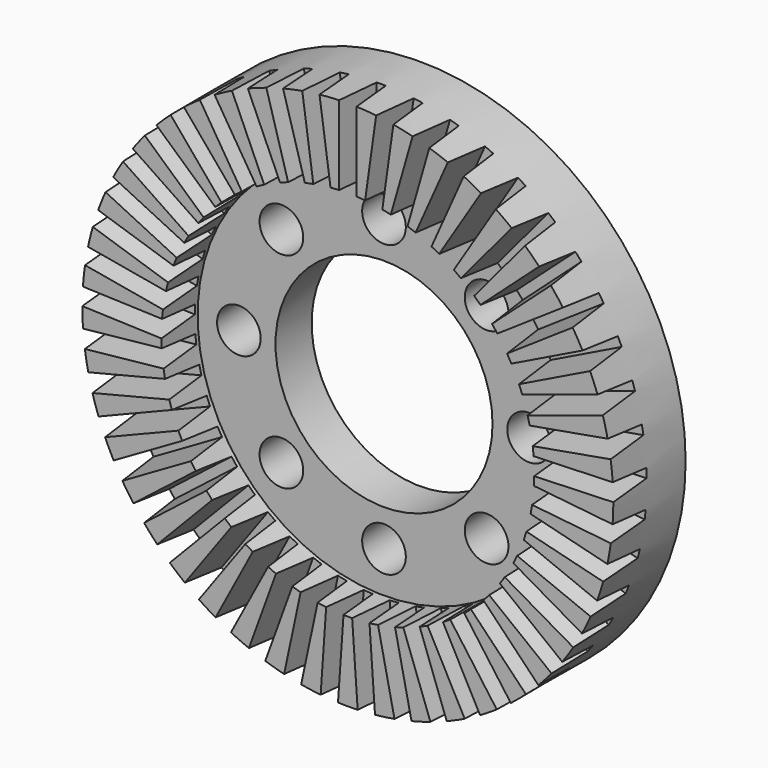
from build123d import *

# Parameters (mm, degrees)
F0_R            = 74.5550854497
F0_R_2          = 30.4767313292
F1_DEPTH        = 25.4
F2_R            = 52.3477403328
F3_DEPTH        = 12.7
F4_R            = 6.1343504353
F5_DEPTH        = 12.7
F8_DEPTH        = 25.4
F8_COPIES_COUNT = 45


# Not quite as in the source:
# - a pattern or mirror of a feature is missing from the dataset's text; its kind, count and spacing are read off the source's solid


with BuildPart() as f1:
    # F0 (on Front) → F1 (new body)
    with BuildSketch(Plane.XZ):
        Circle(F0_R)
        Circle(F0_R_2, mode=Mode.SUBTRACT)
    extrude(amount=F1_DEPTH)

    # F2 (on face) → F3 (cut)
    with BuildSketch(Plane.XZ.offset(25.4)):
        Circle(F2_R)
    extrude(amount=-F3_DEPTH, mode=Mode.SUBTRACT)

    # F4 (on face) → F5 (cut)
    with BuildSketch(Plane.XZ.offset(12.7)):
        with Locations((0, 40.7535322011)):
            Circle(F4_R)
        with Locations((-28.8170989767, 28.8170989767)):
            Circle(F4_R)
        with Locations((-40.7535322011, 0)):
            Circle(F4_R)
        with Locations((-28.8170989767, -28.8170989767)):
            Circle(F4_R)
        with Locations((0, -40.7535322011)):
            Circle(F4_R)
        with Locations((28.8170989767, -28.8170989767)):
            Circle(F4_R)
        with Locations((40.7535322011, 0)):
            Circle(F4_R)
        with Locations((28.8170989767, 28.8170989767)):
            Circle(F4_R)
    extrude(amount=-F5_DEPTH, mode=Mode.SUBTRACT)

    # F7 (on offset) → F8 (cut)
    with BuildSketch(Plane.XY.offset(76.2)):
        Polygon((-1.27, -13.6856001877), (-2.54, -26.3856001877), (2.54, -26.3856001877), (1.27, -13.6856001877), align=None)
    f8 = extrude(amount=-F8_DEPTH, mode=Mode.SUBTRACT)

    # F8_copies: F8 ×45 about axis
    f8_copies_axis = Axis((0, 0, 0), (0, 1, 0))
    for i in range(1, F8_COPIES_COUNT):
        add(f8.rotate(f8_copies_axis, i * 360 / F8_COPIES_COUNT), mode=Mode.SUBTRACT)


solid = f1.part
